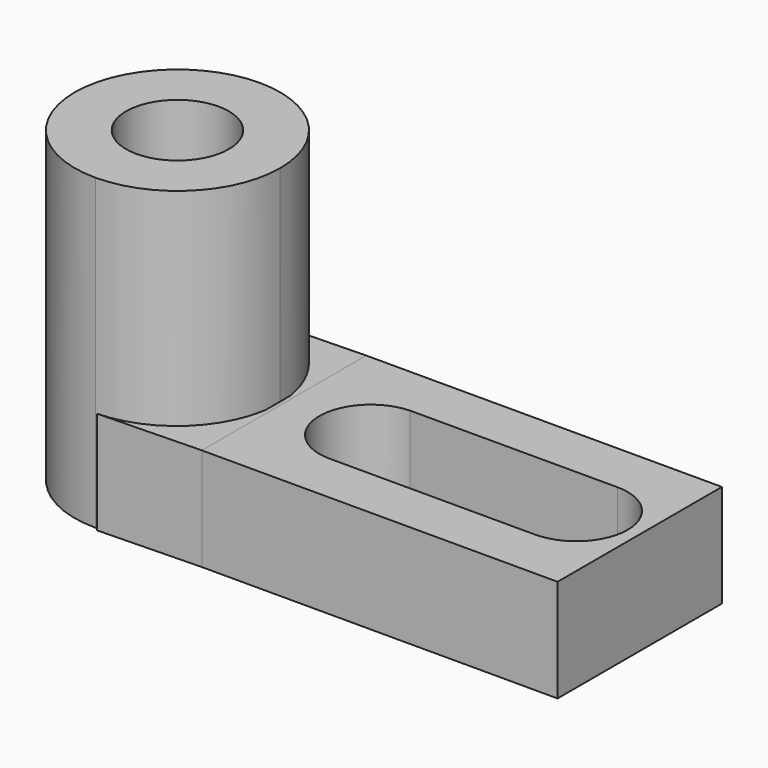
from build123d import *

# Parameters (mm, degrees)
F1_DEPTH = 25.4
F3_DEPTH = 50.8
F4_R     = 6.35
F5_DEPTH = 50.8
F7_DEPTH = 12.7


# Not quite as in the source:
# - a feature names something its author has since deleted; it is built from what else it names


with BuildPart() as f1:
    # F0 (on Front) → F1 (new body)
    with BuildSketch(Plane.XZ):
        Polygon((0, 38.1), (0, 0), (69.85, 0), (69.85, 12.7), (25.4, 12.7), (25.4, 38.1), align=None)
    extrude(amount=F1_DEPTH)

    # F2 (on Top) → F3 (cut)
    with BuildSketch(Plane.XY):
        with BuildLine():
            ThreePointArc((42.9501019467, -12.6976528488), (41.0895425425, -17.1894405959), (36.5977547955, -19.05))
            Line((36.5977547955, -19.05), (61.9977547955, -19.05))
            ThreePointArc((61.9977547955, -19.05), (55.6477547955, -12.7), (61.9977547955, -6.35))
            Line((61.9977547955, -6.35), (36.8419220343, -6.35))
            ThreePointArc((36.8419220343, -6.35), (41.1750547307, -8.2930371297), (42.9501019467, -12.6976528488))
        make_face()
        with BuildLine():
            ThreePointArc((61.9977547955, -6.35), (55.6477547955, -12.7), (61.9977547955, -19.05))
            Line((61.9977547955, -19.05), (61.9977547955, -6.35))
        make_face()
        with BuildLine():
            Line((61.9977547955, -6.35), (61.9977547955, -19.05))
            ThreePointArc((61.9977547955, -19.05), (66.487882856, -17.1901280605), (68.3477547955, -12.7))
            ThreePointArc((68.3477547955, -12.7), (66.487882856, -8.2098719395), (61.9977547955, -6.35))
        make_face()
        with BuildLine():
            Line((36.8419220343, -6.35), (36.3535875566, -6.35))
            Line((36.3535875566, -6.35), (36.5977547955, -19.05))
            ThreePointArc((36.5977547955, -19.05), (41.0895425425, -17.1894405959), (42.9501019467, -12.6976528488))
            ThreePointArc((42.9501019467, -12.6976528488), (41.1750547307, -8.2930371297), (36.8419220343, -6.35))
        make_face()
        with BuildLine():
            Line((36.5977547955, -19.05), (36.3535875566, -6.35))
            ThreePointArc((36.3535875566, -6.35), (30.2465813283, -12.819759029), (36.5977547955, -19.05))
        make_face()
    extrude(amount=F3_DEPTH, mode=Mode.SUBTRACT)

    # F4 (on Top) → F5 (cut)
    with BuildSketch(Plane.XY):
        with BuildLine():
            Line((0, -25.4), (12.7, -25.4))
            ThreePointArc((12.7, -25.4), (3.7197438789, -21.6802561211), (0, -12.7))
            Line((0, -12.7), (0, -25.4))
        make_face()
        with BuildLine():
            Line((0, 0), (0, -12.7))
            ThreePointArc((0, -12.7), (3.7197438789, -3.7197438789), (12.7, 0))
            Line((12.7, 0), (0, 0))
        make_face()
        with BuildLine():
            ThreePointArc((12.7, 0), (21.6802561211, -3.7197438789), (25.4, -12.7))
            Line((25.4, -12.7), (25.4, 0))
            Line((25.4, 0), (12.7, 0))
        make_face()
        with BuildLine():
            ThreePointArc((25.4, -12.7), (21.6802561211, -21.6802561211), (12.7, -25.4))
            Line((12.7, -25.4), (25.4, -25.4))
            Line((25.4, -25.4), (25.4, -12.7))
        make_face()
        with Locations((12.7, -12.7)):
            Circle(F4_R)
    extrude(amount=F5_DEPTH, mode=Mode.SUBTRACT)


with BuildPart() as f7:
    # F6 (on Top) → F7 (new body)
    with BuildSketch(Plane.XY):
        with BuildLine():
            ThreePointArc((13.1827720211, -0.334095074), (25.5529580345, -13.034095074), (13.1827720211, -25.734095074))
            Line((13.1827720211, -25.734095074), (25.8783767913, -25.4))
            Line((25.8783767913, -25.4), (25.8783767913, 0))
            Line((25.8783767913, 0), (13.1827720211, -0.334095074))
        make_face()
    extrude(amount=F7_DEPTH)


solid = Compound([f1.part, f7.part])
